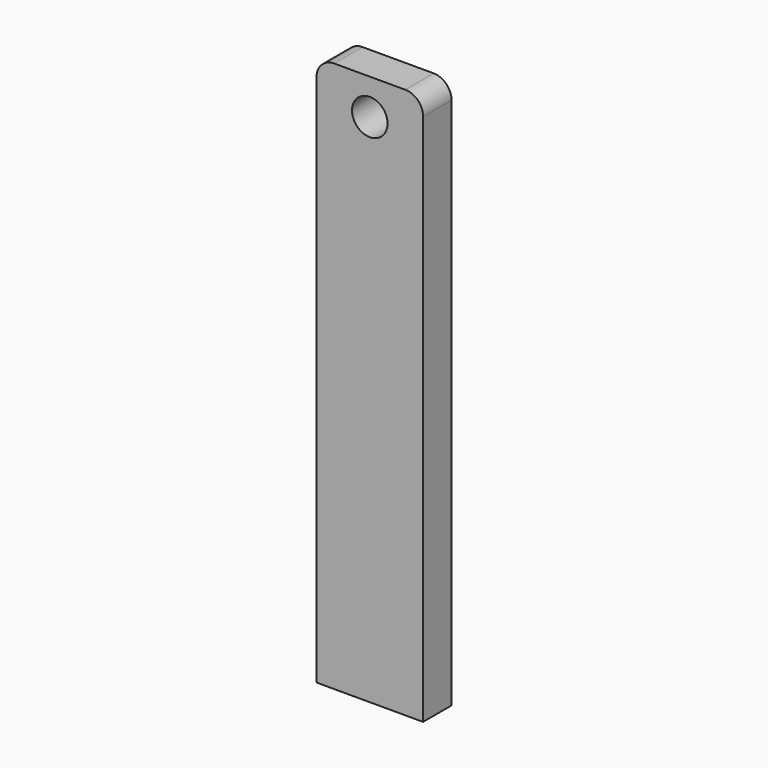
from build123d import *

# Parameters (mm, degrees)
F0_W     = 30
F0_H     = 155
F1_DEPTH = 10
F2_R     = 5
F3_DEPTH = 10.001
F4_R     = 5


# Not quite as in the source:
# - a feature names something its author has since deleted; it is built from what else it names


with BuildPart() as f1:
    # F0 (on Front) → F1 (new body)
    with BuildSketch(Plane.XZ):
        Rectangle(F0_W, F0_H)
    extrude(amount=F1_DEPTH)

    # F2 (on face) → F3 (cut, through all)
    with BuildSketch(Plane.XZ.offset(10)):
        with Locations((0, 67.5)):
            Circle(F2_R)
    extrude(amount=-F3_DEPTH, mode=Mode.SUBTRACT)

    # F4
    f4_edges = [f1.edges().sort_by_distance(p)[0] for p in [
        (15, -5, 77.5),
        (-15, -5, 77.5),
    ]]
    fillet(f4_edges, radius=F4_R)


solid = f1.part
